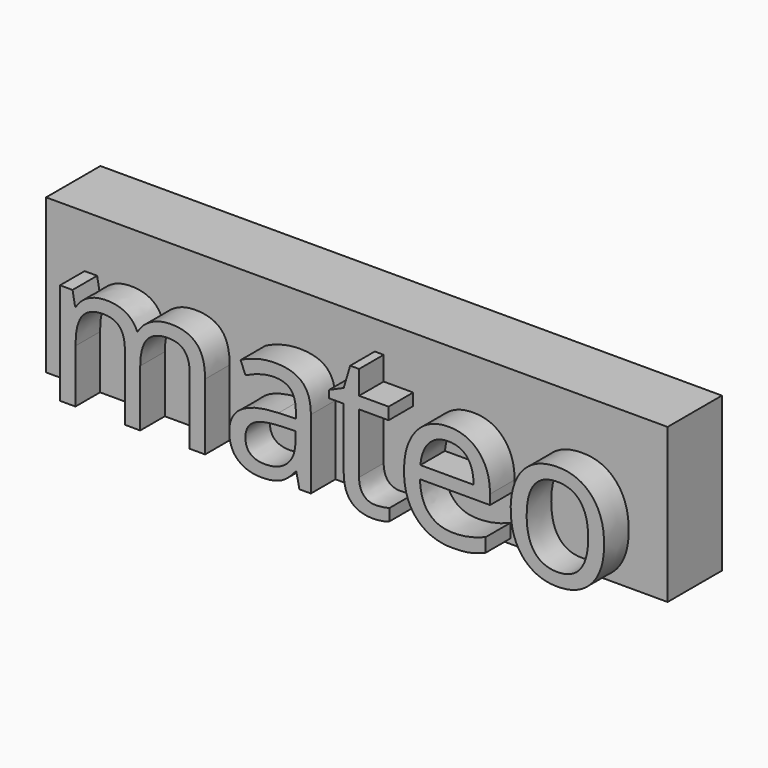
from build123d import *

# Parameters (mm, degrees)
F0_TEXT_SIZE = 22.3863430114
F1_DEPTH     = 3.61869
F2_W         = 73.1851886958
F2_H         = 18.1510895491
F3_DEPTH     = 7.99801


# Not quite as in the source:
# - Text() gives the source's letters only with a copy of the font that has no kerning and outlines rounded to 1/6400 em; it was checked with that copy


with BuildPart() as f1:
    # F0 (on Front) → F1 (new body)
    with BuildSketch(Plane.XZ):
        with Locations((-27.2992383689, 0)):
            Text('mateo', F0_TEXT_SIZE, font='Open Sans', text_align=(TextAlign.LEFT, TextAlign.BOTTOM))
    extrude(amount=F1_DEPTH)


with BuildPart() as f3:
    # F2 (on Front) → F3 (new body)
    with BuildSketch(Plane.XZ):
        with Locations((6.6796028987, 9.0755447745)):
            Rectangle(F2_W, F2_H)
    extrude(amount=-F3_DEPTH)


solid = Compound([f1.part, f3.part])
